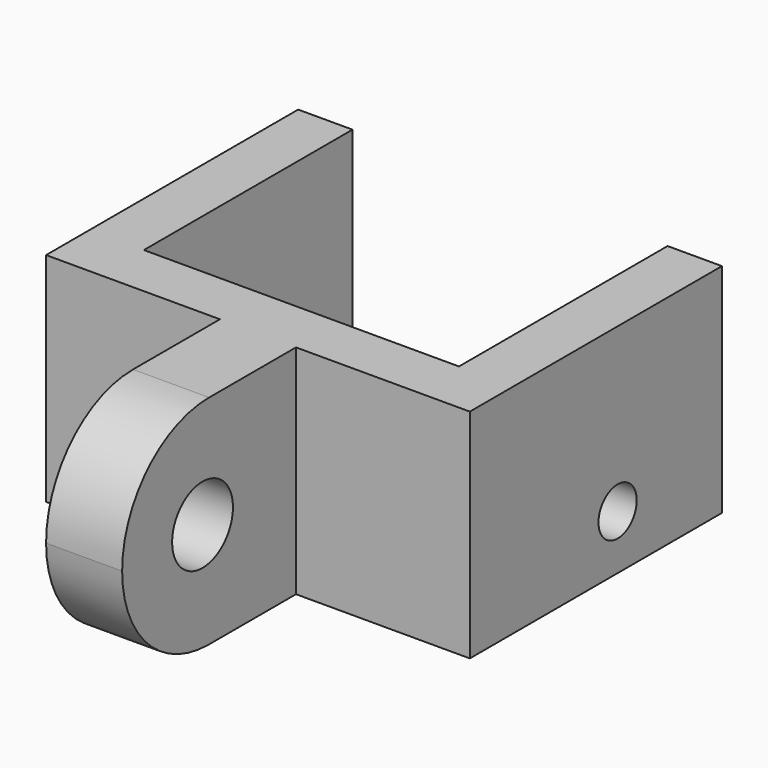
from build123d import *

# Parameters (mm, degrees)
F1_DEPTH = 20
F2_R     = 9.99999
F4_D     = 7
F5_D     = 4.4
F5_DEPTH = 10
F5_TIP   = 1.3218933619


# Not quite as in the source:
# - a fillet or chamfer is up to 0.001 mm smaller than in the source, because OpenCascade refuses the exact size


with BuildPart() as f1:
    # F0 (on Top) → F1 (new body)
    with BuildSketch(Plane.XY):
        Polygon((-18, 49), (-23, 49), (-23, 20), (-7, 20), (-7, 0), (0, 0), (0, 20), (16, 20), (16, 49), (11, 49), (11, 25), (-18, 25), align=None)
    extrude(amount=F1_DEPTH)

    # F2 (radius 10 in the source; OpenCascade refuses exactly that, so slightly less here)
    f2_edges = [f1.edges().sort_by_distance(p)[0] for p in [
        (-3.5, 0, 20),
        (-3.5, 0, 0),
    ]]
    fillet(f2_edges, radius=F2_R)

    # F4 (through all)
    with Locations(Plane.YZ.offset(16)):
        with Locations((9.25, 10)):
            Hole(F4_D / 2)

    # F5
    with Locations(Plane.YZ.offset(16)):
        with Locations((37, 5)):
            Hole(F5_D / 2, depth=F5_DEPTH)
            with Locations((0, 0, -(F5_DEPTH + F5_TIP / 2))):  # 118° drill point
                Cone(0, F5_D / 2, F5_TIP, mode=Mode.SUBTRACT)


solid = f1.part
